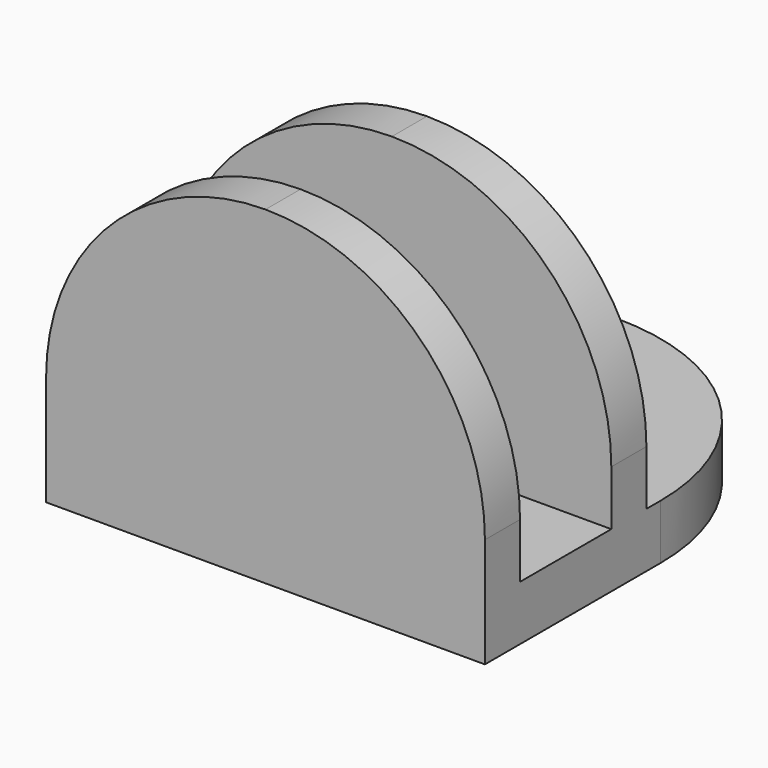
from build123d import *

# Parameters (mm, degrees)
F0_W     = 25.4
F0_H     = 6.604
F1_DEPTH = 3.175
F0_H_2   = 13.716
F0_H_3   = 2.54
F2_DEPTH = 19.05
F3_R     = 12.69999
F4_R     = 1.5875
F5_DEPTH = 25.4
F6_R     = 1.5875
F7_DEPTH = 2.54


# Not quite as in the source:
# - a fillet or chamfer is up to 0.001 mm smaller than in the source, because OpenCascade refuses the exact size


with BuildPart() as f1:
    # F0 (on Top) → F1 (new body)
    with BuildSketch(Plane.XY):
        Rectangle(F0_W, F0_H)
    extrude(amount=F1_DEPTH)



with BuildPart() as f1b:
    # F0 (on Top) → F1, piece 2 (new body)
    with BuildSketch(Plane.XY):
        with Locations((0, 12.7)):
            Rectangle(F0_W, F0_H_2)
    extrude(amount=F1_DEPTH)


with BuildPart() as f1_1:
    add(f1.part)

    add(f1b.part)  # F2 merges F1b
    # F0 (on Top) → F2 (join)
    with BuildSketch(Plane.XY):
        with Locations((0, -4.572)):
            Rectangle(F0_W, F0_H_3)
        with Locations((0, 4.572)):
            Rectangle(F0_W, F0_H_3)
    extrude(amount=F2_DEPTH)

    # F3 (radius 12.7 in the source; OpenCascade refuses exactly that, so slightly less here)
    f3_edges = [f1_1.edges().sort_by_distance(p)[0] for p in [
        (12.7, -4.572, 19.05),
        (12.7, 4.572, 19.05),
        (-12.7, -4.572, 19.05),
        (-12.7, 4.572, 19.05),
        (12.7, 19.558, 1.5875),
        (-12.7, 19.558, 1.5875),
    ]]
    fillet(f3_edges, radius=F3_R)

    # F4 (on face) → F5 (cut)
    with BuildSketch(Plane.XY.offset(3.175)):
        with Locations((0, 12.7)):
            Circle(F4_R)
    extrude(amount=-F5_DEPTH, mode=Mode.SUBTRACT)

    # F6 (on face) → F7 (cut, through all)
    with BuildSketch(Plane(origin=(0, 5.842, 0), x_dir=(-1, 0, 0), z_dir=(0, 1, 0))):
        with Locations((0, 10.033)):
            Circle(F6_R)
    extrude(amount=-F7_DEPTH, mode=Mode.SUBTRACT)


solid = f1_1.part
